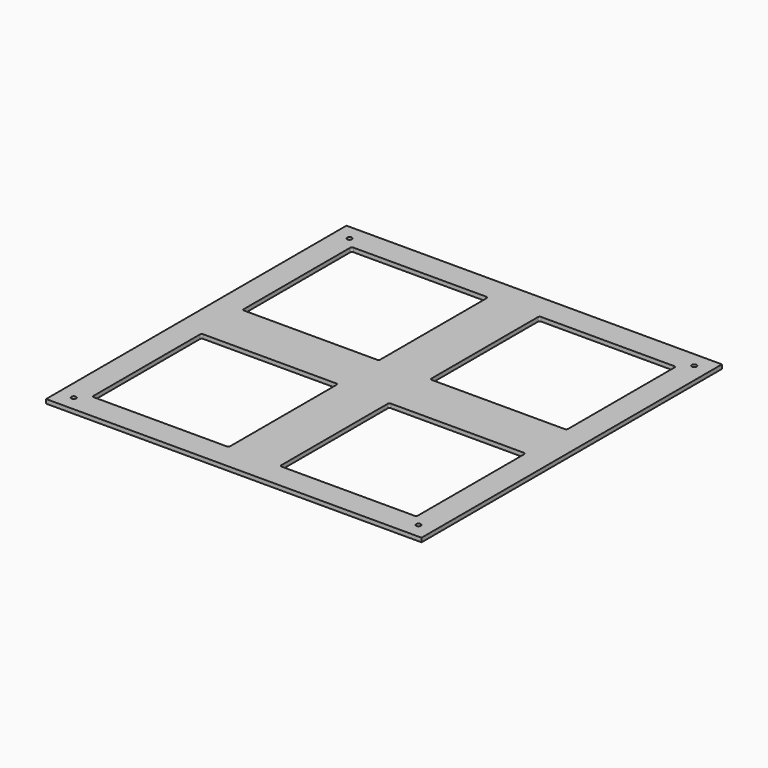
from build123d import *

# Parameters (mm, degrees)
F0_W     = 1100
F0_H     = 1100
F1_DEPTH = 12
F2_R     = 7
F3_DEPTH = 25
F5_DEPTH = 25


# Not quite as in the source:
# - a feature names something its author has since deleted; it is built from what else it names


with BuildPart() as f1:
    # F0 (on Top) → F1 (new body)
    with BuildSketch(Plane.XY):
        Rectangle(F0_W, F0_H)
    extrude(amount=-F1_DEPTH)

    # F2 (on Top) → F3 (cut)
    with BuildSketch(Plane.XY):
        with Locations((-505, -505)):
            Circle(F2_R)
        with Locations((505, 505)):
            Circle(F2_R)
        with Locations((-505, 505)):
            Circle(F2_R)
        with Locations((505, -505)):
            Circle(F2_R)
    extrude(amount=-F3_DEPTH, mode=Mode.SUBTRACT)

    # F4 (on Top) → F5 (cut)
    with BuildSketch(Plane.XY):
        with BuildLine():
            Line((-80, 475), (-470, 475))
            ThreePointArc((-470, 475), (-473.5355339059, 473.5355339059), (-475, 470))
            Line((-475, 470), (-475, 80))
            ThreePointArc((-475, 80), (-473.5355339059, 76.4644660941), (-470, 75))
            Line((-470, 75), (-80, 75))
            ThreePointArc((-80, 75), (-76.4644660941, 76.4644660941), (-75, 80))
            Line((-75, 80), (-75, 470))
            ThreePointArc((-75, 470), (-76.4644660941, 473.5355339059), (-80, 475))
        make_face()
        with BuildLine():
            ThreePointArc((80, 475), (76.4644660941, 473.5355339059), (75, 470))
            Line((75, 470), (75, 80))
            ThreePointArc((75, 80), (76.4644660941, 76.4644660941), (80, 75))
            Line((80, 75), (470, 75))
            ThreePointArc((470, 75), (473.5355339059, 76.4644660941), (475, 80))
            Line((475, 80), (475, 470))
            ThreePointArc((475, 470), (473.5355339059, 473.5355339059), (470, 475))
            Line((470, 475), (80, 475))
        make_face()
        with BuildLine():
            ThreePointArc((475, -80), (473.5355339059, -76.4644660941), (470, -75))
            Line((470, -75), (80, -75))
            ThreePointArc((80, -75), (76.4644660941, -76.4644660941), (75, -80))
            Line((75, -80), (75, -470))
            ThreePointArc((75, -470), (76.4644660941, -473.5355339059), (80, -475))
            Line((80, -475), (470, -475))
            ThreePointArc((470, -475), (473.5355339059, -473.5355339059), (475, -470))
            Line((475, -470), (475, -80))
        make_face()
        with BuildLine():
            ThreePointArc((-475, -470), (-473.5355339059, -473.5355339059), (-470, -475))
            Line((-470, -475), (-80, -475))
            ThreePointArc((-80, -475), (-76.4644660941, -473.5355339059), (-75, -470))
            Line((-75, -470), (-75, -80))
            ThreePointArc((-75, -80), (-76.4644660941, -76.4644660941), (-80, -75))
            Line((-80, -75), (-470, -75))
            ThreePointArc((-470, -75), (-473.5355339059, -76.4644660941), (-475, -80))
            Line((-475, -80), (-475, -470))
        make_face()
    extrude(amount=-F5_DEPTH, mode=Mode.SUBTRACT)


solid = f1.part
